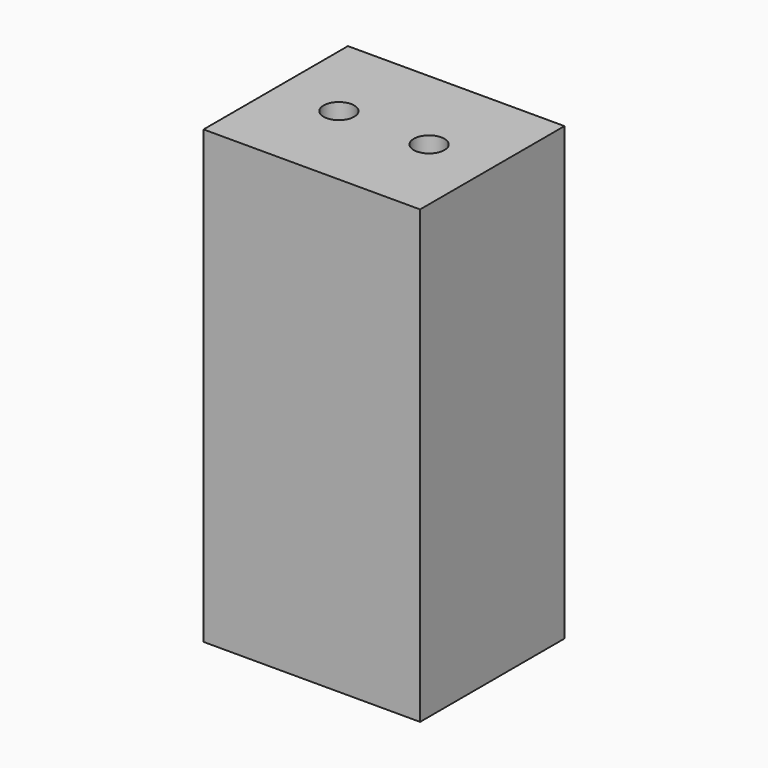
from build123d import *

# Parameters (mm, degrees)
F0_W     = 30.48
F0_H     = 25.4
F0_W_2   = 25.4
F0_H_2   = 20.32
F1_DEPTH = 31.75
F2_W     = 25.4
F2_H     = 20.32
F2_W_2   = 20.32
F2_H_2   = 15.24
F2_R     = 2.159
F3_DEPTH = 12.7
F4_R     = 2.159
F5_DEPTH = 5.08


with BuildPart() as f1:
    # F0 (on Top) → F1 (new body, symmetric)
    with BuildSketch(Plane.XY):
        Rectangle(F0_W, F0_H)
        Rectangle(F0_W_2, F0_H_2, mode=Mode.SUBTRACT)
    extrude(amount=F1_DEPTH, both=True)

    # F2 (on face) → F3 (join)
    with BuildSketch(Plane.XY.offset(31.75)):
        Rectangle(F2_W, F2_H)
        Rectangle(F2_W_2, F2_H_2, mode=Mode.SUBTRACT)
        Rectangle(F2_W_2, F2_H_2)
        with Locations((-6.35, 0)):
            Circle(F2_R, mode=Mode.SUBTRACT)
        with Locations((6.35, 0)):
            Circle(F2_R, mode=Mode.SUBTRACT)
    extrude(amount=-F3_DEPTH)

    # F4 (on face) → F5 (cut)
    with BuildSketch(Plane(origin=(0, 0, 19.05), x_dir=(1, 0, 0), z_dir=(0, 0, -1))):
        Polygon((-3.683, 4.6193795038), (-9.017, 4.6193795038), (-11.684, 0), (-9.017, -4.6193795038), (-3.683, -4.6193795038), (-1.016, 0), align=None)
        with Locations((-6.35, 0)):
            Circle(F4_R, mode=Mode.SUBTRACT)
        Polygon((9.017, 4.6193795038), (3.683, 4.6193795038), (1.016, 0), (3.683, -4.6193795038), (9.017, -4.6193795038), (11.684, 0), align=None)
        with Locations((6.35, 0)):
            Circle(F4_R, mode=Mode.SUBTRACT)
        with Locations((-6.35, 0)):
            Circle(F4_R)
        with Locations((6.35, 0)):
            Circle(F4_R)
    extrude(amount=-F5_DEPTH, mode=Mode.SUBTRACT)


solid = f1.part
